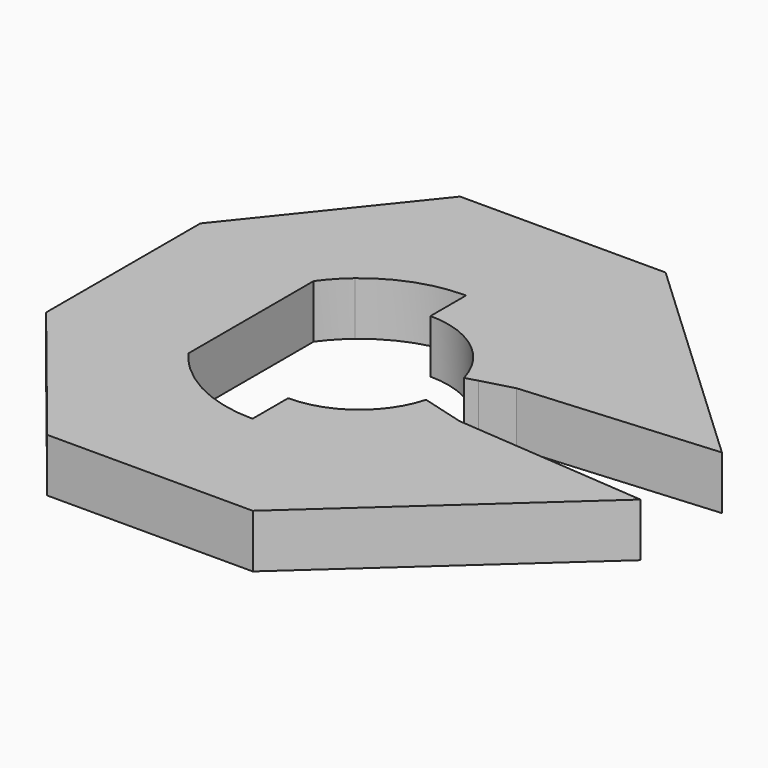
from build123d import *

# Parameters (mm, degrees)
F1_DEPTH = 1.5


# Not quite as in the source:
# - a feature names something its author has since deleted; it is built from what else it names


with BuildPart() as f1:
    # F0 (on Top) → F1 (new body)
    with BuildSketch(Plane.XY):
        with BuildLine():
            ThreePointArc((-4.7637764364, 4.2277344156), (-4.22987066, 3.4988615225), (-3.8857919263, 2.6634449214))
            Line((-3.8857919263, 2.6634449214), (1.5419516712, 3.0945423002))
            Line((1.5419516712, 3.0945423002), (-4.7637764364, 9))
            Line((-4.7637764364, 9), (-4.7637764364, 4.2277344156))
        make_face()
        with BuildLine():
            ThreePointArc((-7.5, -2.0865550786), (-6.0089576806, -1.7773824212), (-4.7637764364, -0.9008445729))
            Line((-4.7637764364, -0.9008445729), (-4.7637764364, 0.9063707553))
            Line((-4.7637764364, 0.9063707553), (-5.0905279509, 0.9967782547))
            ThreePointArc((-5.0905279509, 0.9967782547), (-5.986174823, -0.326111143), (-7.5, -0.8365550786))
            Line((-7.5, -0.8365550786), (-7.5, -2.0865550786))
        make_face()
        with BuildLine():
            Line((-4.7637764364, 2.4205190875), (-4.7637764364, 4.2277344156))
            ThreePointArc((-4.7637764364, 4.2277344156), (-6.0089576806, 5.104272264), (-7.5, 5.4134449214))
            Line((-7.5, 5.4134449214), (-7.5, 4.1634449214))
            ThreePointArc((-7.5, 4.1634449214), (-5.986174823, 3.6530009858), (-5.0905279509, 2.330111588))
            Line((-5.0905279509, 2.330111588), (-4.7637764364, 2.4205190875))
        make_face()
        with BuildLine():
            Line((-10.5388853699, 1.6634449214), (-10.5388853699, 3.8606421607))
            ThreePointArc((-10.5388853699, 3.8606421607), (-11.0677948468, 2.8181483168), (-11.25, 1.6634449214))
            Line((-11.25, 1.6634449214), (-10.5388853699, 1.6634449214))
        make_face()
        with BuildLine():
            ThreePointArc((-11.25, 1.6634449214), (-11.0677948468, 0.5087415259), (-10.5388853699, -0.533752318))
            Line((-10.5388853699, -0.533752318), (-10.5388853699, 1.6634449214))
            Line((-10.5388853699, 1.6634449214), (-11.25, 1.6634449214))
        make_face()
        with BuildLine():
            Line((1.5419516712, 0.2323475426), (-3.8857919263, 0.6634449214))
            ThreePointArc((-3.8857919263, 0.6634449214), (-4.22987066, -0.1719716798), (-4.7637764364, -0.9008445729))
            Line((-4.7637764364, -0.9008445729), (-4.7637764364, -5.4970695637))
            Line((-4.7637764364, -5.4970695637), (1.5419516712, 0.2323475426))
        make_face()
        with BuildLine():
            Line((-4.7637764364, -5.4970695637), (-4.7637764364, -0.9008445729))
            ThreePointArc((-4.7637764364, -0.9008445729), (-6.0089576806, -1.7773824212), (-7.5, -2.0865550786))
            ThreePointArc((-7.5, -2.0865550786), (-8.8586144698, -1.831789938), (-10.0326275495, -1.102110664))
            ThreePointArc((-10.0326275495, -1.102110664), (-10.300213716, -0.8308091044), (-10.5388853699, -0.533752318))
            Line((-10.5388853699, -0.533752318), (-10.5388853699, -5.4970695637))
            Line((-10.5388853699, -5.4970695637), (-4.7637764364, -5.4970695637))
        make_face()
        with BuildLine():
            ThreePointArc((-7.5, 5.4134449214), (-6.0089576806, 5.104272264), (-4.7637764364, 4.2277344156))
            Line((-4.7637764364, 4.2277344156), (-4.7637764364, 9))
            Line((-4.7637764364, 9), (-10.5388853699, 9))
            Line((-10.5388853699, 9), (-10.5388853699, 3.8606421607))
            ThreePointArc((-10.5388853699, 3.8606421607), (-10.2477408327, 4.2153893401), (-9.9154440374, 4.5319166577))
            ThreePointArc((-9.9154440374, 4.5319166577), (-8.7856381662, 5.1861760359), (-7.5, 5.4134449214))
        make_face()
        with BuildLine():
            Line((-10.5388853699, 3.8606421607), (-10.5388853699, 9))
            Line((-10.5388853699, 9), (-14.1904987395, 4.4458052143))
            Line((-14.1904987395, 4.4458052143), (-14.1904987395, -0.9716537897))
            Line((-14.1904987395, -0.9716537897), (-10.5388853699, -5.4970695637))
            Line((-10.5388853699, -5.4970695637), (-10.5388853699, -0.533752318))
            ThreePointArc((-10.5388853699, -0.533752318), (-11.0677948468, 0.5087415259), (-11.25, 1.6634449214))
            ThreePointArc((-11.25, 1.6634449214), (-11.0677948468, 2.8181483168), (-10.5388853699, 3.8606421607))
        make_face()
        with BuildLine():
            ThreePointArc((-4.7637764364, -0.9008445729), (-4.22987066, -0.1719716798), (-3.8857919263, 0.6634449214))
            Line((-3.8857919263, 0.6634449214), (-4.7637764364, 0.9063707553))
            Line((-4.7637764364, 0.9063707553), (-4.7637764364, -0.9008445729))
        make_face()
        with BuildLine():
            Line((-4.7637764364, 2.4205190875), (-3.8857919263, 2.6634449214))
            ThreePointArc((-3.8857919263, 2.6634449214), (-4.22987066, 3.4988615225), (-4.7637764364, 4.2277344156))
            Line((-4.7637764364, 4.2277344156), (-4.7637764364, 2.4205190875))
        make_face()
    extrude(amount=F1_DEPTH)


solid = f1.part
